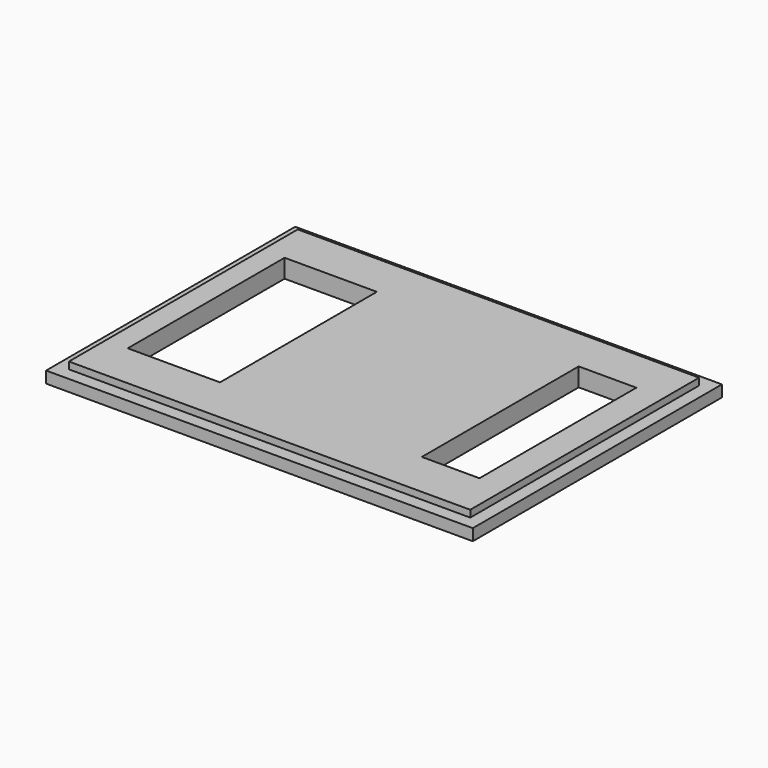
from build123d import *

# Parameters (mm, degrees)
F0_W     = 93.98
F0_H     = 68.58
F1_DEPTH = 2.54
F2_W     = 88.392
F2_H     = 62.992
F3_DEPTH = 1.524
F4_W     = 12.7
F4_H     = 43.18
F5_DEPTH = 4.065
F6_W     = 20.32
F6_H     = 43.18
F7_DEPTH = 4.065


# Not quite as in the source:
# - a feature names something its author has since deleted; it is built from what else it names


with BuildPart() as f1:
    # F0 (on Top) → F1 (new body)
    with BuildSketch(Plane.XY):
        with Locations((-1.1547841132, -14.7677313863)):
            Rectangle(F0_W, F0_H)
    extrude(amount=F1_DEPTH)

    # F2 (on face) → F3 (join)
    with BuildSketch(Plane.XY.offset(2.54)):
        with Locations((-1.1547841132, -14.7677313863)):
            Rectangle(F2_W, F2_H)
    extrude(amount=F3_DEPTH)

    # F4 (on face) → F5 (cut, through all)
    with BuildSketch(Plane.XY.offset(4.064)):
        with Locations((30.5952158868, -14.5137313863)):
            Rectangle(F4_W, F4_H)
    extrude(amount=-F5_DEPTH, mode=Mode.SUBTRACT)

    # F6 (on face) → F7 (cut, through all)
    with BuildSketch(Plane.XY.offset(4.064)):
        with Locations((-30.3647841132, -14.5137313863)):
            Rectangle(F6_W, F6_H)
    extrude(amount=-F7_DEPTH, mode=Mode.SUBTRACT)


solid = f1.part
